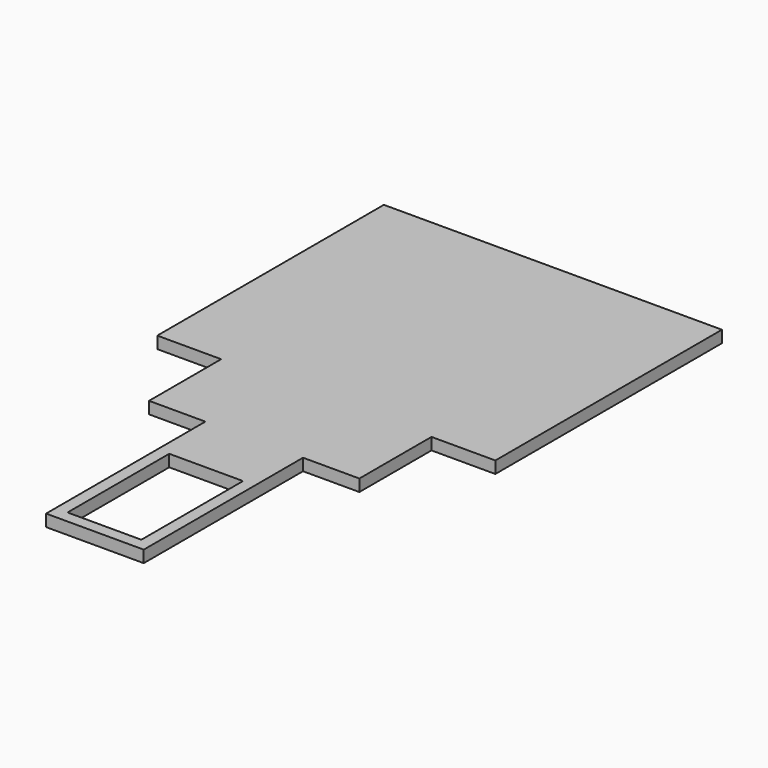
from build123d import *

# Parameters (mm, degrees)
F0_W     = 3.175
F0_H     = 25.4
F0_H_2   = 33.8328
F0_H_3   = 3.175
F1_DEPTH = 3.175
F2_DEPTH = 25.4


# Not quite as in the source:
# - a length typed as a fraction of an inch, garbled in the dataset ("3 / 203.2 mm" for 3/8 in), is restored


with BuildPart() as f1:
    # F0 (on Top) → F1 (new body)
    with BuildSketch(Plane.XY):
        Polygon((-13.825, 0), (0, 0), (56, 0), (69.825, 0), (69.825, 25.4), (-13.825, 25.4), align=None)
        Polygon((56, 0), (0, 0), (0, -23), (0, -50), (0, -74), (15, -74), (28, -74), (41, -74), (56, -74), (56, -50), (56, -23), align=None)
        Polygon((0, -23), (0, 0), (-13.825, 0), (-17, 0), (-17, -50), (0, -50), align=None)
        Polygon((69.825, 0), (56, 0), (56, -23), (56, -50), (73, -50), (73, 0), align=None)
        with Locations((-15.4125, 12.7)):
            Rectangle(F0_W, F0_H)
        with Locations((71.4125, 12.7)):
            Rectangle(F0_W, F0_H)
        Polygon((28, -74), (15, -74), (15, -90), (18.175, -90), (21.35, -90), (28, -90), (34.65, -90), (37.825, -90), (41, -90), (41, -74), align=None)
        with Locations((16.5875, -106.9164)):
            Rectangle(F0_W, F0_H_2)
        with Locations((39.4125, -106.9164)):
            Rectangle(F0_W, F0_H_2)
        with Locations((16.5875, -125.4203)):
            Rectangle(F0_W, F0_H_3)
        with Locations((39.4125, -125.4203)):
            Rectangle(F0_W, F0_H_3)
        Polygon((21.35, -123.8328), (18.175, -123.8328), (18.175, -127.0078), (37.825, -127.0078), (37.825, -123.8328), (34.65, -123.8328), align=None)
    extrude(amount=F1_DEPTH)

    # F0 (on Top) → F2 (cut)
    with BuildSketch(Plane.XY):
        Polygon((28, -90), (21.35, -90), (21.35, -123.8328), (34.65, -123.8328), (34.65, -90), align=None)
    extrude(amount=-F2_DEPTH, mode=Mode.SUBTRACT)


solid = f1.part
